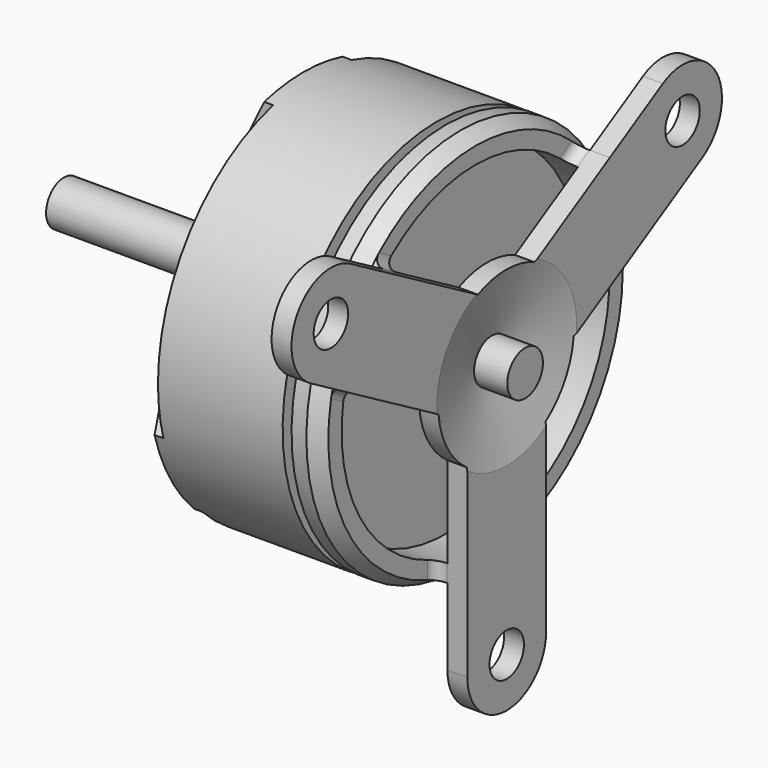
from build123d import *

# Parameters (mm, degrees)
F4_DEPTH = 1.3
F6_DEPTH = 1.05
F5_R     = 0.725
F7_DEPTH = 0.67
F8_R     = 0.3621320344
F8_2_R   = 0.3621320344


# Not quite as in the source:
# - a fillet or chamfer that OpenCascade refuses, or shapes differently, is made with other operations: its cross-section is extruded or revolved along the edge and cut away or added


with BuildPart() as f1:
    # F0 (on Front) → F1 (revolve)
    with BuildSketch(Plane.XZ):
        Polygon((-8.85, 2), (-8.85, 0.75), (-2.35, 0.75), (-2.35, 6.5), (-7.85, 6.5), (-7.85, 2), align=None)
    revolve(axis=Axis((6.5496404592, 0, 0), (1, 0, 0)))

    # F3: chamfer of 2 x 1 on 1 edges, made by hand

    # F3_s1 → F3_t2 (revolve, cut)
    with BuildSketch(Plane.XZ):
        Polygon((-6.85, 6.5), (-7.85, 4.5), (-7.85, 6.5), align=None)
    revolve(axis=Axis((-7.85, 0, 0), (1, 0, 0)), mode=Mode.SUBTRACT)

    # F2 (on face) → F4 (cut)
    with BuildSketch(Plane(origin=(-7.85, 0, 0), x_dir=(0, -1, 0), z_dir=(-1, 0, 0))):
        with BuildLine():
            Line((-1.65, 2.2843407316), (-1.65, 6.2870899469))
            ThreePointArc((-1.65, 6.2870899469), (-5.6291651246, 3.25), (-6.2697796099, -1.7146030572))
            Line((-6.2697796099, -1.7146030572), (-2.8032971045, 0.2867715504))
            ThreePointArc((-2.8032971045, 0.2867715504), (-1.9590250278, 1.1310436271), (-1.65, 2.2843407316))
        make_face()
        with BuildLine():
            ThreePointArc((6.5, 0), (5.14660082, 3.9702015062), (1.65, 6.2870899469))
            Line((1.65, 6.2870899469), (1.65, 2.2843407316))
            ThreePointArc((1.65, 2.2843407316), (1.9590250278, 1.1310436271), (2.8032971045, 0.2867715504))
            Line((2.8032971045, 0.2867715504), (6.2697796099, -1.7146030572))
            ThreePointArc((6.2697796099, -1.7146030572), (6.4421878063, -0.8649949526), (6.5, 0))
        make_face()
        with BuildLine():
            Line((-1.1532971045, -2.571112282), (-4.6197796099, -4.5724868897))
            ThreePointArc((-4.6197796099, -4.5724868897), (0, -6.5), (4.6197796099, -4.5724868897))
            Line((4.6197796099, -4.5724868897), (1.1532971045, -2.571112282))
            ThreePointArc((1.1532971045, -2.571112282), (0, -2.2620872543), (-1.1532971045, -2.571112282))
        make_face()
    extrude(amount=-F4_DEPTH, mode=Mode.SUBTRACT)

    # F8
    f8_edges = [f1.edges().sort_by_distance(p)[0] for p in [
        (-7.85, 0, 4.5),
        (-7.85, 3.897114, -2.25),
        (-7.85, -3.897114, -2.25),
        (-8.85, 0, -2),
    ]]
    fillet(f8_edges, radius=F8_R)



with BuildPart() as f1b:
    # F0 (on Front) → F1, piece 2 (revolve)
    with BuildSketch(Plane.XZ):
        Polygon((-0.67, 0.75), (0, 0.75), (0, 6.2), (-1.05, 6.2), (-1.55, 6.5), (-2.05, 6.5), (-2.05, 5.64), (-0.67, 5.64), align=None)
    revolve(axis=Axis((6.5496404592, 0, 0), (1, 0, 0)))

    # F5 (on face) → F6 (cut)
    with BuildSketch(Plane.YZ):
        with BuildLine():
            ThreePointArc((4.3433258161, 4.4244232228), (0, 6.2), (-4.3433258161, 4.4244232228))
            Line((-4.3433258161, 4.4244232228), (-1.1869283577, 2.6020763005))
            ThreePointArc((-1.1869283577, 2.6020763005), (0, 2.86), (1.1869283577, 2.6020763005))
            Line((1.1869283577, 2.6020763005), (4.3433258161, 4.4244232228))
        make_face()
        with BuildLine():
            Line((1.66, -2.3289482605), (1.66, -5.9736421051))
            ThreePointArc((1.66, -5.9736421051), (4.936192865, -3.75153302), (6.2, 0))
            ThreePointArc((6.2, 0), (6.150634929, 0.780826466), (6.0033258161, 1.5492188823))
            Line((6.0033258161, 1.5492188823), (2.8469283577, -0.27312804))
            ThreePointArc((2.8469283577, -0.27312804), (2.4768326548, -1.43), (1.66, -2.3289482605))
        make_face()
        with BuildLine():
            ThreePointArc((-6.0033258161, 1.5492188823), (-5.3693575035, -3.1), (-1.66, -5.9736421051))
            Line((-1.66, -5.9736421051), (-1.66, -2.3289482605))
            ThreePointArc((-1.66, -2.3289482605), (-2.4768326548, -1.43), (-2.8469283577, -0.27312804))
            Line((-2.8469283577, -0.27312804), (-6.0033258161, 1.5492188823))
        make_face()
    extrude(amount=-F6_DEPTH, mode=Mode.SUBTRACT)

    # F5 (on face) → F7 (join)
    with BuildSketch(Plane.YZ):
        with BuildLine():
            Line((-8.2345172024, 2.8373978297), (-6.0033258161, 1.5492188823))
            ThreePointArc((-6.0033258161, 1.5492188823), (-5.3693575035, 3.1), (-4.3433258161, 4.4244232228))
            Line((-4.3433258161, 4.4244232228), (-6.5745172024, 5.7126021703))
            ThreePointArc((-6.5745172024, 5.7126021703), (-8.8421193726, 5.105), (-8.2345172024, 2.8373978297))
        make_face()
        with Locations((-7.4045172024, 4.275)):
            Circle(F5_R, mode=Mode.SUBTRACT)
        with BuildLine():
            ThreePointArc((4.3433258161, 4.4244232228), (5.3693575035, 3.1), (6.0033258161, 1.5492188823))
            Line((6.0033258161, 1.5492188823), (8.2345172024, 2.8373978297))
            ThreePointArc((8.2345172024, 2.8373978297), (8.8421193726, 5.105), (6.5745172024, 5.7126021703))
            Line((6.5745172024, 5.7126021703), (4.3433258161, 4.4244232228))
        make_face()
        with Locations((7.4045172024, 4.275)):
            Circle(F5_R, mode=Mode.SUBTRACT)
        with BuildLine():
            Line((1.66, -8.55), (1.66, -5.9736421051))
            ThreePointArc((1.66, -5.9736421051), (0, -6.2), (-1.66, -5.9736421051))
            Line((-1.66, -5.9736421051), (-1.66, -8.55))
            ThreePointArc((-1.66, -8.55), (0, -10.21), (1.66, -8.55))
        make_face()
        with Locations((0, -8.55)):
            Circle(F5_R, mode=Mode.SUBTRACT)
    extrude(amount=-F7_DEPTH)

    # F8#2
    f8_2_edges = [f1b.edges().sort_by_distance(p)[0] for p in [
        (-1.05, -5.750678, 1.403352),
        (-1.05, -4.090678, 4.278557),
        (-1.05, 4.090678, 4.278557),
        (-1.05, 5.750678, 1.403352),
        (-1.05, 1.66, -5.681909),
        (-1.05, -1.66, -5.681909),
    ]]
    fillet(f8_2_edges, radius=F8_2_R)

    # F9: chamfer of 2.2 x 0.5 on 1 edges, made by hand

    # F9_s1 → F9_t2 (revolve, cut)
    with BuildSketch(Plane.XZ):
        Polygon((0, 2.95), (-0.5, 0.75), (0, 0.75), align=None)
    revolve(axis=Axis((0, 0, 0), (1, 0, 0)), mode=Mode.SUBTRACT)


with BuildPart() as f1_1:
    add(f1.part)

    add(f1b.part)  # F10 merges F1b
    # F0 (on Front) → F10 (revolve)
    with BuildSketch(Plane.XZ):
        Polygon((-14.92, 0.75), (-14.92, 0), (0.62, 0), (0.62, 0.75), (0, 0.75), (-0.67, 0.75), (-2.35, 0.75), (-8.85, 0.75), align=None)
    revolve(axis=Axis((6.5496404592, 0, 0), (1, 0, 0)))


solid = f1_1.part
